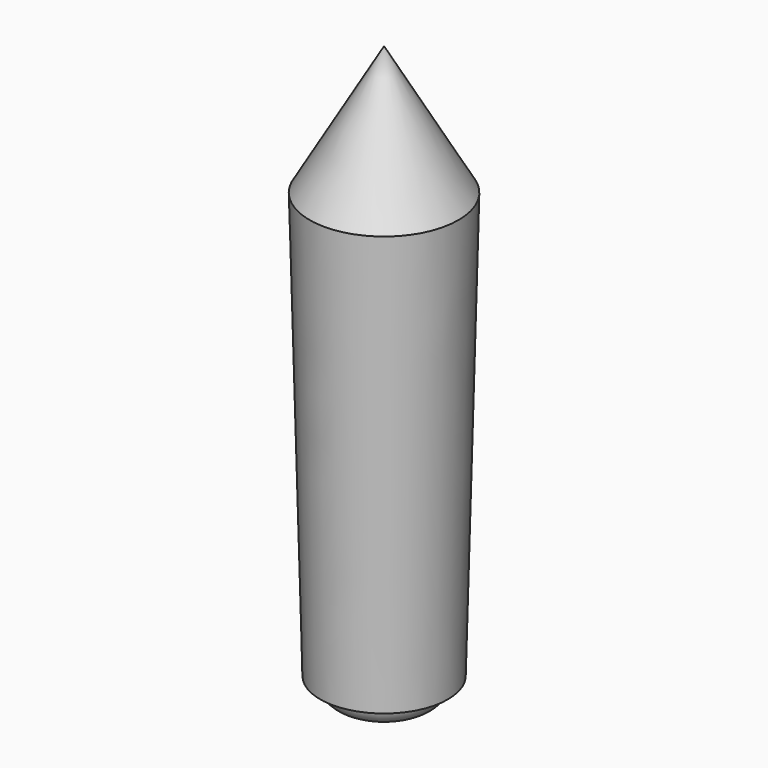
from build123d import *

# Parameters (mm, degrees)
F2_R = 3.99999


# Not quite as in the source:
# - a fillet or chamfer is up to 0.001 mm smaller than in the source, because OpenCascade refuses the exact size


with BuildPart() as f1:
    # F0 (on Front) → F1 (revolve)
    with BuildSketch(Plane.XZ):
        Polygon((14, -24.248711306), (0, 0), (0, -108.248711306), (10, -108.248711306), (10, -104.248711306), (12, -104.248711306), align=None)
    revolve(axis=Axis((0, 0, -54.124355653), (0, 0, 1)))

    # F2 (radius 4 in the source; OpenCascade refuses exactly that, so slightly less here)
    f2_edges = [f1.edges().sort_by_distance(p)[0] for p in [
        (-10, 0, -108.248711),
    ]]
    fillet(f2_edges, radius=F2_R)


solid = f1.part
